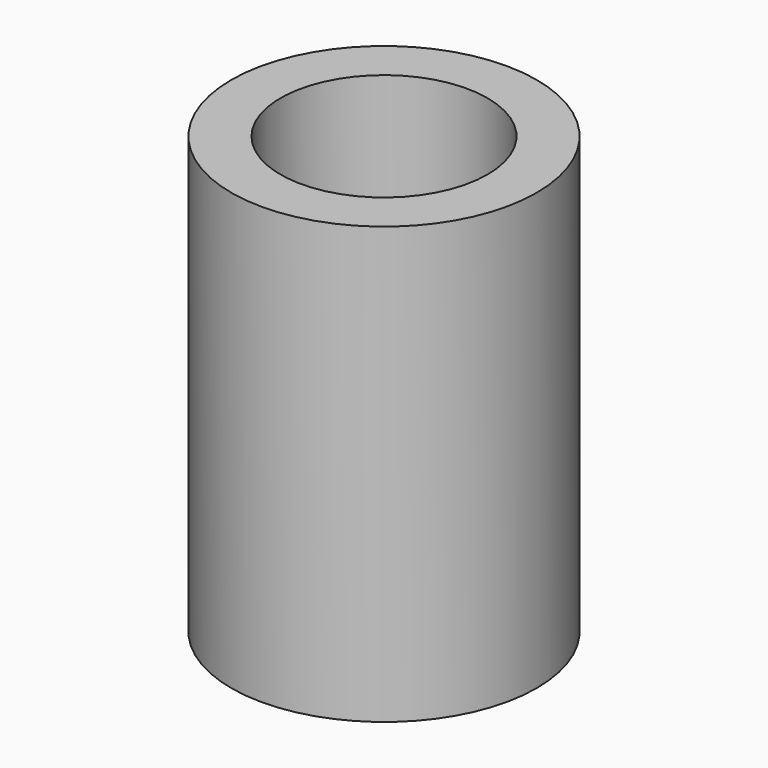
from build123d import *

# Parameters (mm, degrees)
F0_R     = 37.2630205799
F1_DEPTH = 106.4
F3_DEPTH = 86.5
F5_R     = 25.2537141006
F6_DEPTH = 102.8


# Not quite as in the source:
# - a feature names something its author has since deleted; it is built from what else it names


with BuildPart() as f1:
    # F0 (on Top) → F1 (new body)
    with BuildSketch(Plane.XY):
        Circle(F0_R)
    extrude(amount=F1_DEPTH)

    # F2 (on face) → F3 (join)
    with BuildSketch(Plane.XY.offset(106.4)):
        Polygon((4.5720788687, -32.5187220476), (30.4480788261, -12.2998245754), (25.8759999575, 20.2188974722), (-4.5720788687, 32.5187220476), (-30.4480788261, 12.2998245754), (-25.8759999575, -20.2188974722), align=None)
    extrude(amount=-F3_DEPTH)

    # F5 (on face) → F6 (cut)
    with BuildSketch(Plane.XY.offset(106.4)):
        Circle(F5_R)
    extrude(amount=-F6_DEPTH, mode=Mode.SUBTRACT)


solid = f1.part
